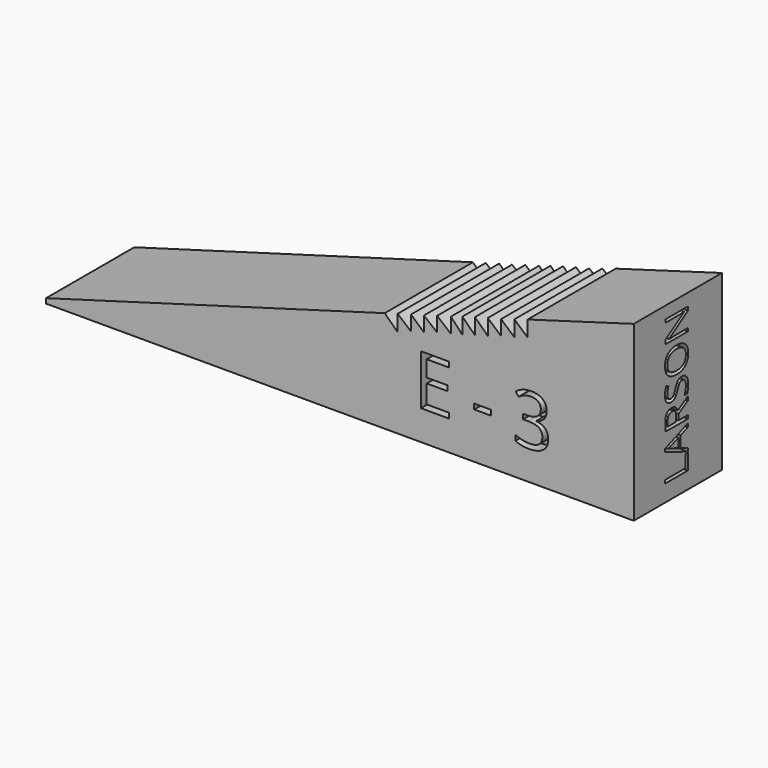
from build123d import *

# Parameters (mm, degrees)
F1_DEPTH     = 25
F2_TEXT_SIZE = 15.9423552557
F4_DEPTH     = 3
F3_TEXT_SIZE = 15.9423552557
F5_DEPTH     = 3
F6_TEXT_SIZE = 8.9658883394
F7_DEPTH     = 2


# Not quite as in the source:
# - Text() gives the source's letters only with a copy of the font that has no kerning and outlines rounded to 1/6400 em; it was checked with that copy


with BuildPart() as f1:
    # F0 (on Front) → F1 (new body)
    with BuildSketch(Plane.XZ):
        Polygon((-59.0122230351, -21.3820207864), (-57.9569935799, -21.3575270027), (74.3279606104, -21.3575270027), (74.3279606104, 17.9704297334), (50.2419397235, 11.0080651939), (50.2419397235, 7.432796061), (47.231182456, 10.0672040135), (47.231182456, 6.4919358119), (44.2204326391, 9.1263446957), (44.2204326391, 5.7392474264), (41.2096790969, 8.3736563101), (41.2096790969, 4.7983871773), (38.2793433964, 7.5989789329), (38.2793433964, 3.9946706966), (35.4294255376, 6.760767661), (35.4294255376, 3.1564596575), (32.8309722245, 5.9225563891), (32.8309722245, 2.4858908728), (29.7295898199, 5.0843455829), (29.7295898199, 1.7315007281), (26.7120301723, 4.1623134166), (26.7120301723, 0.8094683872), (23.7782914191, 3.407923039), (23.7782914191, 0), (20.7607299089, 2.569712), (20.7607299089, -1.11841748), (17.8269911557, 1.7315007281), (-59.0122230351, -20.2563684704), align=None)
    extrude(amount=F1_DEPTH)

    # F2 (on face) → F4 (cut)
    with BuildSketch(Plane.XZ.offset(25)):
        with Locations((24.4623702019, -14.5833347924)):
            Text('E - 3', F2_TEXT_SIZE, font='Open Sans', text_align=(TextAlign.LEFT, TextAlign.BOTTOM))
    extrude(amount=-F4_DEPTH, mode=Mode.SUBTRACT)

    # F3 (on face) → F5 (cut)
    with BuildSketch(Plane(origin=(0, 0, 0), x_dir=(-1, 0, 0), z_dir=(0, 1, 0))):
        with Locations((-55.9475468472, -14.8470071144)):
            Text('E - 3', F3_TEXT_SIZE, font='Open Sans', text_align=(TextAlign.LEFT, TextAlign.BOTTOM))
    extrude(amount=-F5_DEPTH, mode=Mode.SUBTRACT)

    # F6 (on face) → F7 (cut)
    with BuildSketch(Plane.YZ.offset(74.3279606104)):
        with Locations(Location((-9.6908602864, -18.4408612549), (0, 0, 89.883672674))):
            Text('LARSON', F6_TEXT_SIZE, font='Open Sans', text_align=(TextAlign.LEFT, TextAlign.BOTTOM))
    extrude(amount=-F7_DEPTH, mode=Mode.SUBTRACT)


solid = f1.part
